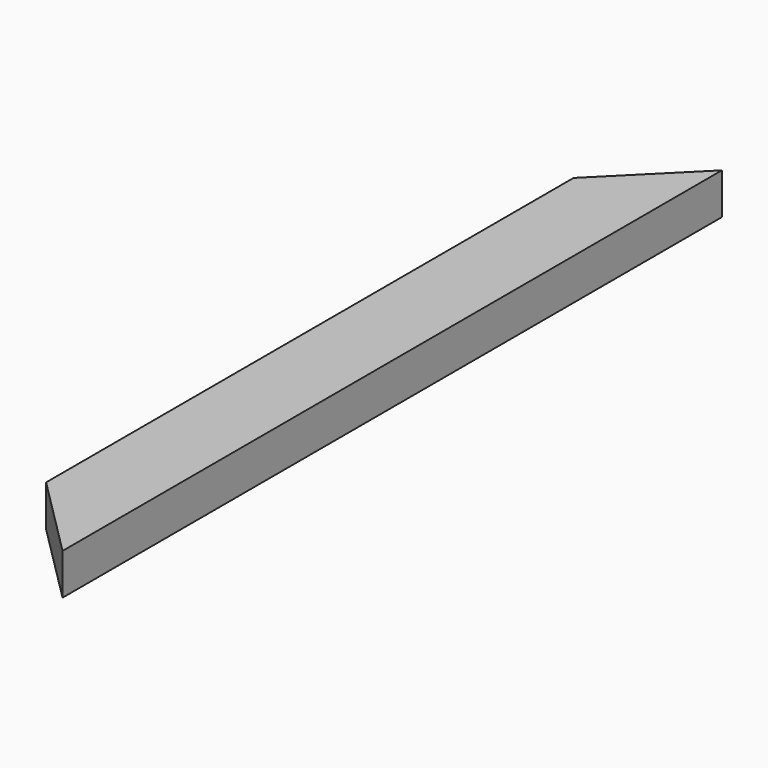
from build123d import *

# Parameters (mm, degrees)
F0_W     = 50.8
F0_H     = 25.4
F1_DEPTH = 508
F2_SIZE  = 50.79999
F3_SIZE  = 50.79999


# Not quite as in the source:
# - a fillet or chamfer is up to 0.001 mm smaller than in the source, because OpenCascade refuses the exact size


with BuildPart() as f1:
    # F0 (on Front) → F1 (new body)
    with BuildSketch(Plane.XZ):
        with Locations((-7.1503547952, 11.2930212758)):
            Rectangle(F0_W, F0_H)
    extrude(amount=F1_DEPTH)

    # F2 (size 50.8 in the source; OpenCascade refuses exactly that, so slightly less here)
    f2_edges = [f1.edges().sort_by_distance(p)[0] for p in [
        (-32.550355, -508, 11.293021),
    ]]
    chamfer(f2_edges, length=F2_SIZE)

    # F3 (size 50.8 in the source; OpenCascade refuses exactly that, so slightly less here)
    f3_edges = [f1.edges().sort_by_distance(p)[0] for p in [
        (-32.550355, 0, 11.293021),
    ]]
    chamfer(f3_edges, length=F3_SIZE)


solid = f1.part
